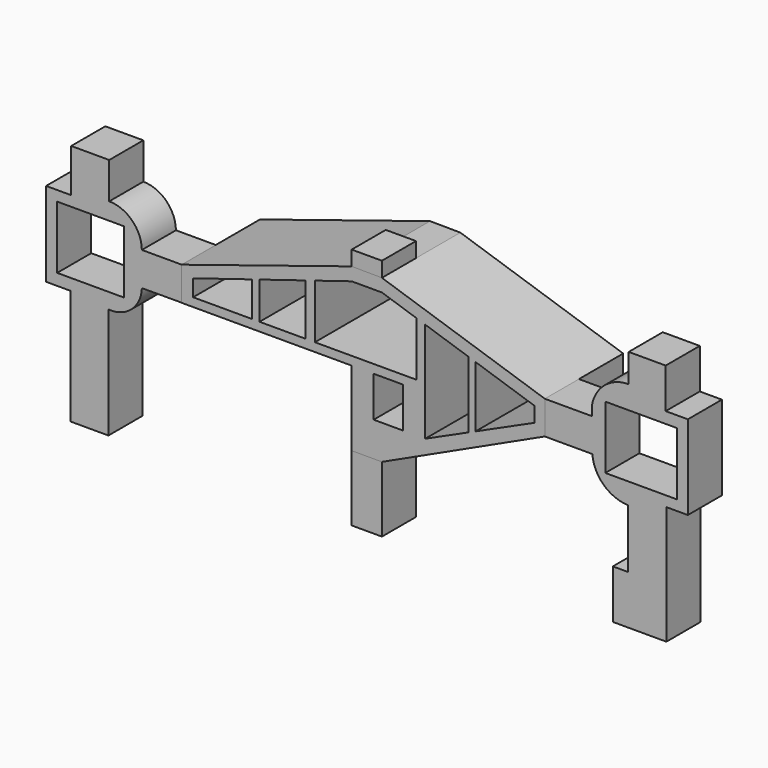
from build123d import *

# Parameters (mm, degrees)
F1_DEPTH = 20
F0_W     = 33.5354409566
F0_H     = 29.4713070616
F0_W_2   = 13.8462930918
F0_H_2   = 18.9892888787
F2_DEPTH = 46


# Not quite as in the source:
# - a feature names something its author has since deleted; it is built from what else it names


with BuildPart() as f1:
    # F0 (on Front) → F1 (new body)
    with BuildSketch(Plane.XZ):
        with BuildLine():
            Line((-155.6314946512, 67.6252768617), (-155.6314946512, 47.2762209197))
            Line((-155.6314946512, 47.2762209197), (-167.4313265361, 47.2762209197))
            Line((-167.4313265361, 47.2762209197), (-167.4313265361, 7.6476708777))
            Line((-167.4313265361, 7.6476708777), (-155.8691086427, 7.6476708777))
            Line((-155.8691086427, 7.6476708777), (-155.8691086427, -46.3575256138))
            Line((-155.8691086427, -46.3575256138), (-138.1710558739, -46.3595552359))
            Line((-138.1710558739, -46.3595552359), (-138.1710558739, 5.7931691183))
            ThreePointArc((-138.1710558739, 5.7931691183), (-127.3375674722, 9.3473401396), (-122.4768718044, 19.6609350621))
            Line((-122.4768718044, 19.6609350621), (-103.9673313431, 19.7311375442))
            Line((-103.9673313431, 19.7311375442), (-103.8078861008, 19.6609350621))
            Line((-103.8078861008, 19.6609350621), (-103.7908970378, 35.4393695202))
            Line((-103.7908970378, 35.4393695202), (-122.4768718044, 35.4393695202))
            ThreePointArc((-122.4768718044, 35.4393695202), (-127.0403675747, 46.1257386332), (-137.7895793309, 50.5391755124))
            Line((-137.7895793309, 50.5391755124), (-137.7895793309, 67.6252768617))
            Line((-137.7895793309, 67.6252768617), (-155.6314946512, 67.6252768617))
        make_face()
        Polygon((-154.9718528986, 42.4946472049), (-130.7401065387, 42.4946472049), (-130.7401065387, 13.0343120545), (-162.2313265361, 13.0343120545), (-162.2313265361, 35.5673134327), (-162.2313265361, 42.4946472049), align=None, mode=Mode.SUBTRACT)
    extrude(amount=-F1_DEPTH)


with BuildPart() as f1b:
    # F0 (on Front) → F1, piece 2 (new body)
    with BuildSketch(Plane.XZ):
        Polygon((-9.785844778, -15.4884296749), (-23.9759656186, -15.4884296749), (-23.9759656186, -46.3726511895), (-9.785844778, -46.3742785201), align=None)
        Polygon((-9.785844778, -46.3742785201), (-23.9759656186, -46.3726511895), (-23.9759656186, -46.3895921645), (-9.785844778, -46.3895921645), align=None)
    extrude(amount=-F1_DEPTH)


with BuildPart() as f1c:
    # F0 (on Front) → F1, piece 3 (new body)
    with BuildSketch(Plane.XZ):
        Polygon((-23.9759656186, 67.6252768617), (-23.9759656186, 60.675183593), (-9.785844778, 60.5657943495), (-9.785844778, 67.6252768617), align=None)
    extrude(amount=-F1_DEPTH)


with BuildPart() as f1d:
    # F0 (on Front) → F1, piece 4 (new body)
    with BuildSketch(Plane.XZ):
        with BuildLine():
            Line((88.7390607463, 35.4548891909), (66.6762858462, 35.4548891909))
            Line((66.6762858462, 35.4548891909), (66.6762858462, 19.8677930884))
            Line((66.6762858462, 19.8677930884), (88.9697274822, 19.8677930884))
            ThreePointArc((88.9697274822, 19.8677930884), (94.3221237474, 8.8416564285), (105.6684866268, 4.2065852498))
            Line((105.6684866268, 4.2065852498), (105.6684866268, -23.4245071926))
            Line((105.6684866268, -23.4245071926), (98.6128924986, -23.4245071926))
            Line((98.6128924986, -23.4245071926), (98.6128924986, -25.1669372239))
            Line((98.6128924986, -25.1669372239), (98.6128924986, -46.3867097448))
            Line((98.6128924986, -46.3867097448), (123.7472345797, -46.3895921645))
            Line((123.7472345797, -46.3895921645), (123.7472345797, -42.8738521096))
            Line((123.7472345797, -42.8738521096), (123.7472345797, 9.2341114881))
            Line((123.7472345797, 9.2341114881), (133.8177919388, 9.2341114881))
            Line((133.8177919388, 9.2341114881), (133.8177919388, 48.7965246565))
            Line((133.8177919388, 48.7965246565), (123.4177919388, 48.7965246565))
            Line((123.4177919388, 48.7965246565), (123.4177919388, 67.6252768617))
            Line((123.4177919388, 67.6252768617), (106.0500037662, 67.6252768617))
            Line((106.0500037662, 67.6252768617), (106.0500037662, 54.2760035917))
            ThreePointArc((106.0500037662, 54.2760035917), (94.7286096073, 50.1405055605), (88.7390607463, 39.6809829085))
            Line((88.7390607463, 39.6809829085), (88.7390607463, 35.4548891909))
        make_face()
        with Locations((111.8500714605, 28.7748654373)):
            Rectangle(F0_W, F0_H, mode=Mode.SUBTRACT)
    extrude(amount=-F1_DEPTH)


with BuildPart() as f2:
    # F0 (on Front) → F2 (new body)
    with BuildSketch(Plane.XZ):
        Polygon((-103.745634354, 35.4393695202), (-103.7908970378, 35.4393695202), (-103.8078861008, 19.6609350621), (-89.1917004483, 19.6609350621), (-23.9759656186, 19.6609350621), (-23.9759656186, -15.4884296749), (-9.785844778, -15.4884296749), (66.6762858462, 19.8677930884), (66.6762858462, 35.4548891909), (-9.785844778, 60.5657943495), (-23.9759656186, 60.675183593), align=None)
        with Locations((-6.7280486905, 10.1662906227)):
            Rectangle(F0_W_2, F0_H_2, mode=Mode.SUBTRACT)
        Polygon((-70.7811092775, 23.7144525419), (-98.4061571746, 23.7144525419), (-98.4061571746, 31.5614215695), (-70.7811092775, 40.0778087067), align=None, mode=Mode.SUBTRACT)
        Polygon((-67.2195533208, 23.7144525419), (-67.2195533208, 41.1757828876), (-45.5977594697, 47.841457015), (-45.5977594697, 23.7144525419), align=None, mode=Mode.SUBTRACT)
        Polygon((-41.2550495299, 49.1802492303), (-23.9759656186, 54.5071311424), (-9.785844778, 54.5071311424), (6.4343885435, 49.1802492303), (6.4343885435, 23.7144525419), (-41.2550495299, 23.7144525419), align=None, mode=Mode.SUBTRACT)
        Polygon((10.5109801516, 47.841457015), (30.8078050811, 41.1757828876), (30.8078050811, 9.8754427638), (10.5109801516, 0.6716461834), align=None, mode=Mode.SUBTRACT)
        Polygon((34.1511112947, 40.0778087067), (61.8842991005, 30.9699608995), (61.8842991005, 23.9673872123), (34.1511112947, 11.3914981273), align=None, mode=Mode.SUBTRACT)
    extrude(amount=-F2_DEPTH)


solid = Compound([f1.part, f1b.part, f1c.part, f1d.part, f2.part])
